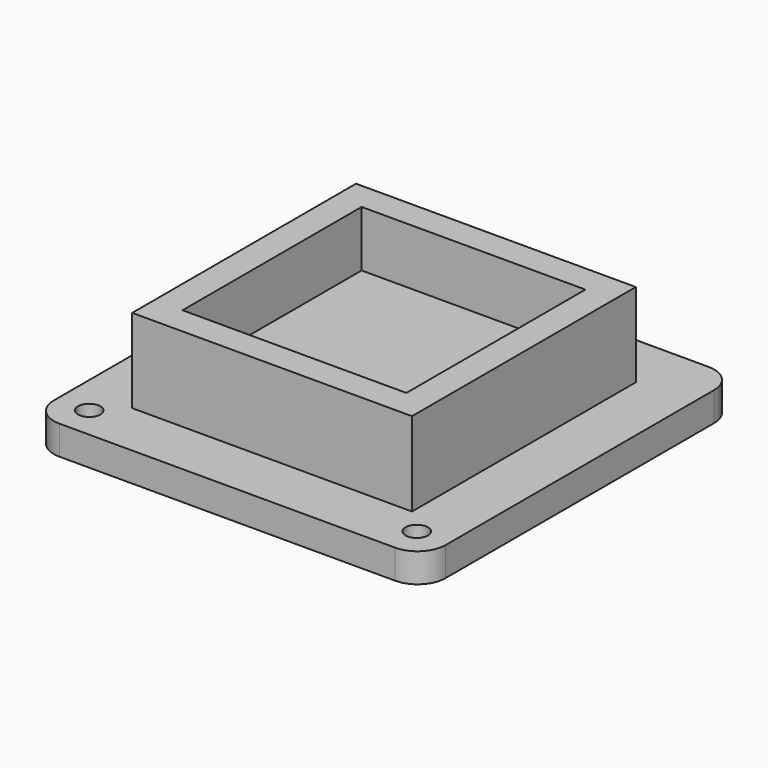
from build123d import *

# Parameters (mm, degrees)
F0_W     = 70
F0_H     = 70
F1_DEPTH = 5.2
F2_W     = 50
F2_H     = 50
F3_DEPTH = 15
F4_R     = 5
F5_R     = 2
F6_DEPTH = 2.7
F8_W     = 40
F8_H     = 40
F9_DEPTH = 10


# Not quite as in the source:
# - a feature names something its author has since deleted; it is built from what else it names


with BuildPart() as f1:
    # F0 (on Top) → F1 (new body)
    with BuildSketch(Plane.XY):
        Rectangle(F0_W, F0_H)
    extrude(amount=F1_DEPTH)

    # F2 (on face) → F3 (join)
    with BuildSketch(Plane.XY.offset(5.2)):
        Rectangle(F2_W, F2_H)
    extrude(amount=F3_DEPTH)

    # F4
    f4_edges = [f1.edges().sort_by_distance(p)[0] for p in [
        (-35, 35, 2.6),
        (35, 35, 2.6),
        (35, -35, 2.6),
        (-35, -35, 2.6),
    ]]
    fillet(f4_edges, radius=F4_R)

    # F5 (on face) → F6 (cut)
    with BuildSketch(Plane.XY.offset(5.2)):
        with Locations((-29, 29)):
            Circle(F5_R)
        with Locations((29.267766953, -29.267766953)):
            Circle(F5_R)
        with Locations((-29.267766953, -29.267766953)):
            Circle(F5_R)
    extrude(amount=-F6_DEPTH, mode=Mode.SUBTRACT)

    # F8 (on face) → F9 (cut)
    with BuildSketch(Plane.XY.offset(20.2)):
        Rectangle(F8_W, F8_H)
    extrude(amount=-F9_DEPTH, mode=Mode.SUBTRACT)


solid = f1.part
